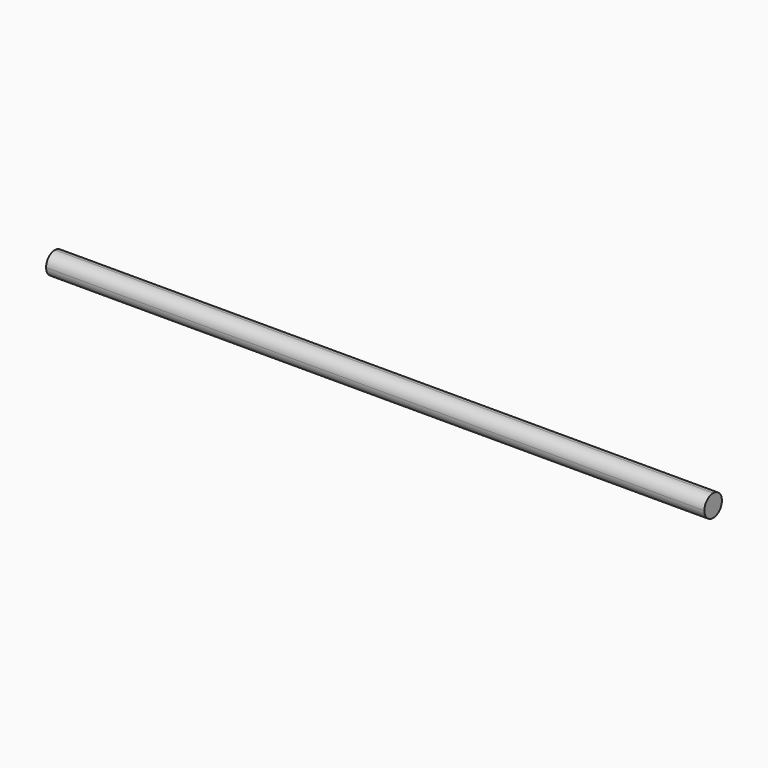
from build123d import *

# Parameters (mm, degrees)
F0_W     = 1200
F0_H     = 40
F1_DEPTH = 40
F2_R     = 19.99999


# Not quite as in the source:
# - a fillet or chamfer is up to 0.001 mm smaller than in the source, because OpenCascade refuses the exact size


with BuildPart() as f1:
    # F0 (on Front) → F1 (new body)
    with BuildSketch(Plane.XZ):
        with Locations((41.1198027432, -62.495377017)):
            Rectangle(F0_W, F0_H)
    extrude(amount=F1_DEPTH)

    # F2 (radius 20 in the source; OpenCascade refuses exactly that, so slightly less here)
    f2_edges = [f1.edges().sort_by_distance(p)[0] for p in [
        (41.119803, -40, -42.495377),
        (41.119803, 0, -42.495377),
        (41.119803, -40, -82.495377),
        (41.119803, 0, -82.495377),
    ]]
    fillet(f2_edges, radius=F2_R)


solid = f1.part
